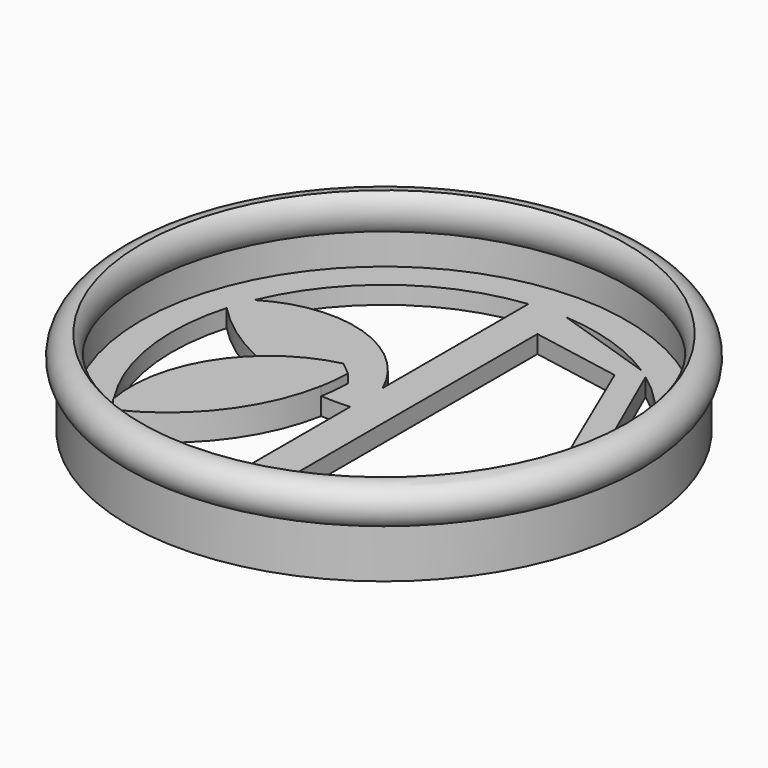
from build123d import *

# Parameters (mm, degrees)
F3_DEPTH = 2
F4_DEPTH = 1


# Not quite as in the source:
# - a feature names something its author has since deleted; it is built from what else it names


with BuildPart() as f1:
    # F0 (on Front) → F1 (revolve)
    with BuildSketch(Plane.XZ):
        Polygon((-29, 0), (-24, 0), (-24, 2), (-27.5, 2), (-27.5, 5.5), (-29, 5.5), align=None)
        with BuildLine():
            ThreePointArc((-27.5, 9.6169896424), (-29.7772258205, 8.1149302096), (-29, 5.5))
            Line((-29, 5.5), (-27.5, 5.5))
            ThreePointArc((-27.5, 5.5), (-26.6610115833, 7.5584948212), (-27.5, 9.6169896424))
        make_face()
    revolve(axis=Axis((0, 0, 2.7132770047), (0, 0, -1)))

    # F2 (on face) → F3 (join)
    with BuildSketch(Plane.XY.offset(2)):
        with BuildLine():
            Line((23.5357220544, -2.0133285341), (14.1158952872, 19.40982999))
            ThreePointArc((14.1158952872, 19.40982999), (13.5624984717, 19.8004705804), (12.9982976167, 20.1753378923))
            Line((12.9982976167, 20.1753378923), (1.5001369464, 23.9530705577))
            ThreePointArc((1.5001369464, 23.9530705577), (-0.61185618, 23.9921993993), (-2.7191094967, 23.8454700844))
            Line((-2.7191094967, 23.8454700844), (-2.7191094967, 3.205855377))
            Line((-2.7191094967, 3.205855377), (-2.7191094967, -1.398249995))
            Line((-2.7191094967, -1.398249995), (-2.7191094967, -23.8454700844))
            ThreePointArc((-2.7191094967, -23.8454700844), (-0.6587764532, -23.9909569127), (1.406435812, -23.9587549407))
            Line((1.406435812, -23.9587549407), (23.3430031088, -5.5771144744))
            ThreePointArc((23.3430031088, -5.5771144744), (23.6412294167, -4.1342800662), (23.8503615327, -2.6758652355))
            Line((23.8503615327, -2.6758652355), (23.5357220544, -2.0133285341))
        make_face()
        Polygon((1.5001369464, -17.0947052702), (1.5001369464, 19.8581963794), (11.7461745714, 17.9819713885), (19.9739150703, -1.2165056542), align=None, mode=Mode.SUBTRACT)
        with BuildLine():
            ThreePointArc((-2.7191094967, 3.205855377), (-11.036038033, 10.667911986), (-22.125575094, 9.2983292455))
            ThreePointArc((-22.125575094, 9.2983292455), (-22.6453594845, 7.9490687392), (-23.0829490937, 6.5709558771))
            ThreePointArc((-23.0829490937, 6.5709558771), (-14.7738683342, 6.6118059769), (-7.1936681304, 3.2084169794))
            ThreePointArc((-7.1936681304, 3.2084169794), (-6.4176007096, 2.6054477842), (-5.6727145132, 1.9643572708))
            ThreePointArc((-5.6727145132, 1.9643572708), (-4.0996738523, 0.3675861057), (-2.7191094967, -1.398249995))
            Line((-2.7191094967, -1.398249995), (-2.7191094967, 3.205855377))
        make_face()
        with BuildLine():
            ThreePointArc((-7.1936681304, 3.2084169794), (-14.7738683342, 6.6118059769), (-23.0829490937, 6.5709558771))
            ThreePointArc((-23.0829490937, 6.5709558771), (-18.5638120771, 2.8268811021), (-13.3236565945, 0.1846347444))
            ThreePointArc((-13.3236565945, 0.1846347444), (-10.4265323426, 2.0368417185), (-7.1936681304, 3.2084169794))
        make_face()
        with BuildLine():
            ThreePointArc((-13.3236565945, 0.1846347444), (-9.7250792571, -0.8614617254), (-6.0139401649, -1.3825407177))
            ThreePointArc((-6.0139401649, -1.3825407177), (-5.7755854856, 0.2840018043), (-5.6727145132, 1.9643572708))
            ThreePointArc((-5.6727145132, 1.9643572708), (-6.4176007096, 2.6054477842), (-7.1936681304, 3.2084169794))
            ThreePointArc((-7.1936681304, 3.2084169794), (-10.4265323426, 2.0368417185), (-13.3236565945, 0.1846347444))
        make_face()
        with BuildLine():
            ThreePointArc((-18.8341819929, -14.8752676836), (-18.1973718669, -15.6478642996), (-17.528892227, -16.3932283976))
            ThreePointArc((-17.528892227, -16.3932283976), (-9.9671253359, -10.2719865524), (-6.0139401649, -1.3825407177))
            ThreePointArc((-6.0139401649, -1.3825407177), (-9.7250792571, -0.8614617254), (-13.3236565945, 0.1846347444))
            ThreePointArc((-13.3236565945, 0.1846347444), (-18.1653516525, -6.5818760317), (-18.8341819929, -14.8752676836))
        make_face()
        with BuildLine():
            ThreePointArc((-6.0139401649, -1.3825407177), (-4.3667724447, -1.4423293633), (-2.7191094967, -1.398249995))
            ThreePointArc((-2.7191094967, -1.398249995), (-4.0996738523, 0.3675861057), (-5.6727145132, 1.9643572708))
            ThreePointArc((-5.6727145132, 1.9643572708), (-5.7755854856, 0.2840018043), (-6.0139401649, -1.3825407177))
        make_face()
    extrude(amount=-F3_DEPTH)

    # F2 (on face) → F4 (join)
    with BuildSketch(Plane.XY.offset(2)):
        with BuildLine():
            ThreePointArc((-18.8341819929, -14.8752676836), (-18.1973718669, -15.6478642996), (-17.528892227, -16.3932283976))
            ThreePointArc((-17.528892227, -16.3932283976), (-9.9671253359, -10.2719865524), (-6.0139401649, -1.3825407177))
            ThreePointArc((-6.0139401649, -1.3825407177), (-9.7250792571, -0.8614617254), (-13.3236565945, 0.1846347444))
            ThreePointArc((-13.3236565945, 0.1846347444), (-18.1653516525, -6.5818760317), (-18.8341819929, -14.8752676836))
        make_face()
        with BuildLine():
            ThreePointArc((-13.3236565945, 0.1846347444), (-9.7250792571, -0.8614617254), (-6.0139401649, -1.3825407177))
            ThreePointArc((-6.0139401649, -1.3825407177), (-5.7755854856, 0.2840018043), (-5.6727145132, 1.9643572708))
            ThreePointArc((-5.6727145132, 1.9643572708), (-6.4176007096, 2.6054477842), (-7.1936681304, 3.2084169794))
            ThreePointArc((-7.1936681304, 3.2084169794), (-10.4265323426, 2.0368417185), (-13.3236565945, 0.1846347444))
        make_face()
    extrude(amount=F4_DEPTH)


solid = f1.part
